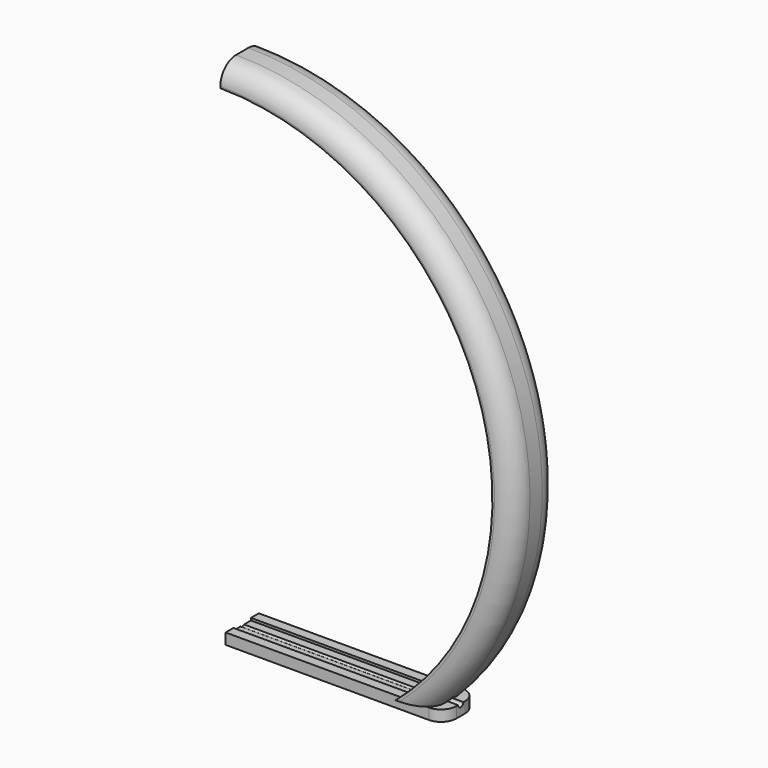
from build123d import *

# Parameters (mm, degrees)
F1_DEPTH     = 12.5
F3_DEPTH     = 145
F4_W         = 200
F4_H         = 19
F5_DEPTH     = 5
F7_DEPTH     = 5
F8_R         = 1
F9_DEPTH     = 135.4900855741
F11_T3_ANGLE = 288.8835060345
F11_T7_ANGLE = 288.8835060345
F12_W        = 164.3678992987
F12_H        = 299.086984247
F13_DEPTH    = 15
F14_R        = 1.5
F15_DEPTH    = 3
F16_R        = 1.5
F17_DEPTH    = 3
F18_SIZE     = 0.5
F19_R        = 1.5
F20_DEPTH    = 134.5119145259
F21_R        = 7


# Not quite as in the source:
# - a fillet or chamfer that OpenCascade refuses, or shapes differently, is made with other operations: its cross-section is extruded or revolved along the edge and cut away or added


with BuildPart() as f1:
    # F0 (on Front) → F1 (new body, symmetric)
    with BuildSketch(Plane.XZ):
        with BuildLine():
            ThreePointArc((95.206740787, 0), (-0.4890855741, 230.2224176182), (-96.1849119353, 0))
            Line((-96.1849119353, 0), (95.206740787, 0))
        make_face()
    extrude(amount=F1_DEPTH, both=True)

    # F2 (on face) → F3 (cut, symmetric)
    with BuildSketch(Plane.XZ.offset(12.5)):
        with BuildLine():
            ThreePointArc((80.206740787, 0), (-0.4890855741, 220.4629960136), (-81.1849119353, 0))
            Line((-81.1849119353, 0), (80.206740787, 0))
        make_face()
    extrude(amount=F3_DEPTH, both=True, mode=Mode.SUBTRACT)

    # F4 (on Top) → F5 (join)
    with BuildSketch(Plane.XY):
        Rectangle(F4_W, F4_H)
    extrude(amount=-F5_DEPTH)

    # F6 (on Front) → F7 (cut, symmetric)
    with BuildSketch(Plane.XZ):
        with BuildLine():
            ThreePointArc((86.5775826458, -1.0740190898), (-0.4890855741, 225.4629960136), (-87.5557537941, -1.0740190898))
            Line((-87.5557537941, -1.0740190898), (86.5775826458, -1.0740190898))
        make_face()
    extrude(amount=F7_DEPTH, both=True, mode=Mode.SUBTRACT)

    # F8 (on Right) → F9 (cut, through all)
    with BuildSketch(Plane.YZ):
        Circle(F8_R)
    extrude(amount=-F9_DEPTH, mode=Mode.SUBTRACT)

    # F11: fillet of radius 9 on 2 edges, made by hand


with BuildPart() as f11_tool1:
    # F11_s2 → F11_t3 (revolve)
    with BuildSketch(Plane(origin=(44.7250174756, 0, 31.9706955431), x_dir=(0, 1, 0), z_dir=(-0.8135247542, 0, -0.5815302867))):
        with BuildLine():
            ThreePointArc((-12.5, 48.2497880385), (-9.8639610307, 54.6137490692), (-3.5, 57.2497880385))
            Line((-3.5, 57.2497880385), (-3.5, 57.4297880385))
            Line((-3.5, 57.4297880385), (-12.68, 57.4297880385))
            Line((-12.68, 57.4297880385), (-12.68, 48.2497880385))
            Line((-12.68, 48.2497880385), (-12.5, 48.2497880385))
        make_face()
    revolve(axis=Axis((-0.4890855741, -12.5, 95.2224176182), (0, -1, 0)), revolution_arc=F11_T3_ANGLE)

    split(bisect_by=Plane.XY, keep=Keep.TOP)


with BuildPart() as f11_tool5:
    # F11_s6 → F11_t7 (revolve)
    with BuildSketch(Plane(origin=(44.7250174756, 0, 31.9706955431), x_dir=(0, 1, 0), z_dir=(-0.8135247542, 0, -0.5815302867))):
        with BuildLine():
            ThreePointArc((3.5, 57.2497880385), (9.8639610307, 54.6137490692), (12.5, 48.2497880385))
            Line((12.5, 48.2497880385), (12.68, 48.2497880385))
            Line((12.68, 48.2497880385), (12.68, 57.4297880385))
            Line((12.68, 57.4297880385), (3.5, 57.4297880385))
            Line((3.5, 57.4297880385), (3.5, 57.2497880385))
        make_face()
    revolve(axis=Axis((-0.4890855741, 12.5, 95.2224176182), (0, -1, 0)), revolution_arc=F11_T7_ANGLE)

    split(bisect_by=Plane.XY, keep=Keep.TOP)


with BuildPart() as f1_1:
    add(f1.part)

    # F11_t9: cut F11_tool1, F11_tool5
    add([f11_tool1.part, f11_tool5.part], mode=Mode.SUBTRACT)

    # F12 (on Front) → F13 (cut, symmetric)
    with BuildSketch(Plane.XZ):
        with Locations((-82.1839496493, 121.752621606)):
            Rectangle(F12_W, F12_H)
    extrude(amount=F13_DEPTH, both=True, mode=Mode.SUBTRACT)

    # F14 (on face) → F15 (join)
    with BuildSketch(Plane(origin=(0, 0, 0), x_dir=(0, -1, 0), z_dir=(-1, 0, 0))):
        with Locations((-8.75, 225.4620759923)):
            Circle(F14_R)
    extrude(amount=F15_DEPTH)

    # F16 (on face) → F17 (cut)
    with BuildSketch(Plane(origin=(0, 0, 0), x_dir=(0, -1, 0), z_dir=(-1, 0, 0))):
        with Locations((8.75, 225.4620759923)):
            Circle(F16_R)
    extrude(amount=-F17_DEPTH, mode=Mode.SUBTRACT)

    # F18
    f18_edges = [f1_1.edges().sort_by_distance(p)[0] for p in [
        (-3, 10.25, 225.462076),
    ]]
    chamfer(f18_edges, length=F18_SIZE)

    # F19 (on Right) → F20 (cut, through all)
    with BuildSketch(Plane.YZ):
        Circle(F19_R)
    extrude(amount=F20_DEPTH, mode=Mode.SUBTRACT)

    # F21
    f21_edges = [f1_1.edges().sort_by_distance(p)[0] for p in [
        (100, 9.5, -2.5),
        (100, -9.5, -2.5),
    ]]
    fillet(f21_edges, radius=F21_R)


solid = f1_1.part
